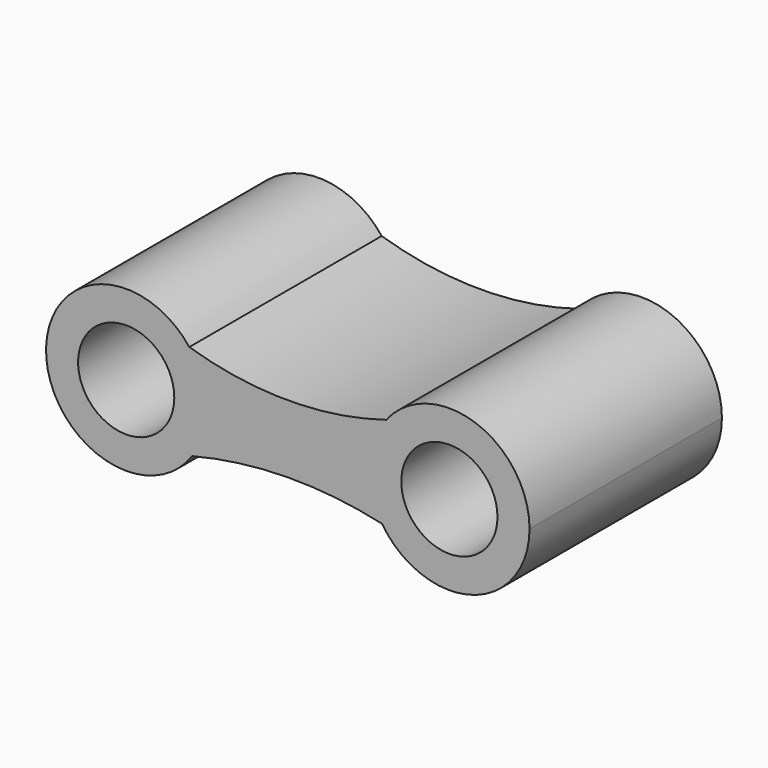
from build123d import *

# Parameters (mm, degrees)
F0_R     = 15.24
F1_DEPTH = 76.2
F2_R     = 15.24
F3_DEPTH = 12.7


# Not quite as in the source:
# - the program builds the solid bodies; features that only make, move or delete a surface that nothing else refers to are left out


with BuildPart() as f1:
    # F0 (on Front) → F1 (new body)
    with BuildSketch(Plane.XZ):
        with BuildLine():
            ThreePointArc((-30.7586478548, -14.4772019242), (-27.3878303212, -7.5846439713), (-26.2289766602, 0))
            ThreePointArc((-26.2289766602, 0), (-27.6162300636, 8.2793720106), (-31.6264570452, 15.6543670921))
            ThreePointArc((-31.6264570452, 15.6543670921), (-77.0184488356, -0.7312336534), (-30.7586478548, -14.4772019242))
        make_face()
        with Locations((-51.6289766602, 0)):
            Circle(F0_R, mode=Mode.SUBTRACT)
        with BuildLine():
            ThreePointArc((-31.6264570452, 15.6543670921), (-27.6162300636, 8.2793720106), (-26.2289766602, 0))
            ThreePointArc((-26.2289766602, 0), (-27.3878303212, -7.5846439713), (-30.7586478548, -14.4772019242))
            ThreePointArc((-30.7586478548, -14.4772019242), (-0.6990994055, -10.5436994312), (29.4432734756, -13.7819477124))
            ThreePointArc((29.4432734756, -13.7819477124), (25.4048776906, 1.1438261277), (30.7698211259, 15.6457138385))
            ThreePointArc((30.7698211259, 15.6457138385), (-0.4289690246, 10.9553864554), (-31.6264570452, 15.6543670921))
        make_face()
        with BuildLine():
            ThreePointArc((76.179109931, 0), (59.0532885715, 24.014536594), (30.7698211259, 15.6457138385))
            ThreePointArc((30.7698211259, 15.6457138385), (25.4048776906, 1.1438261277), (29.4432734756, -13.7819477124))
            ThreePointArc((29.4432734756, -13.7819477124), (57.9634593807, -24.3627815116), (76.179109931, 0))
        make_face()
        with Locations((50.779109931, 0)):
            Circle(F0_R, mode=Mode.SUBTRACT)
    extrude(amount=F1_DEPTH)

    # F2 (on Front) → F3 (join)
    with BuildSketch(Plane.XZ):
        with Locations((-51.3377061976, 0)):
            Circle(F2_R)
        with Locations((50.8029804159, 0)):
            Circle(F2_R)
    extrude(amount=F3_DEPTH)


solid = f1.part
